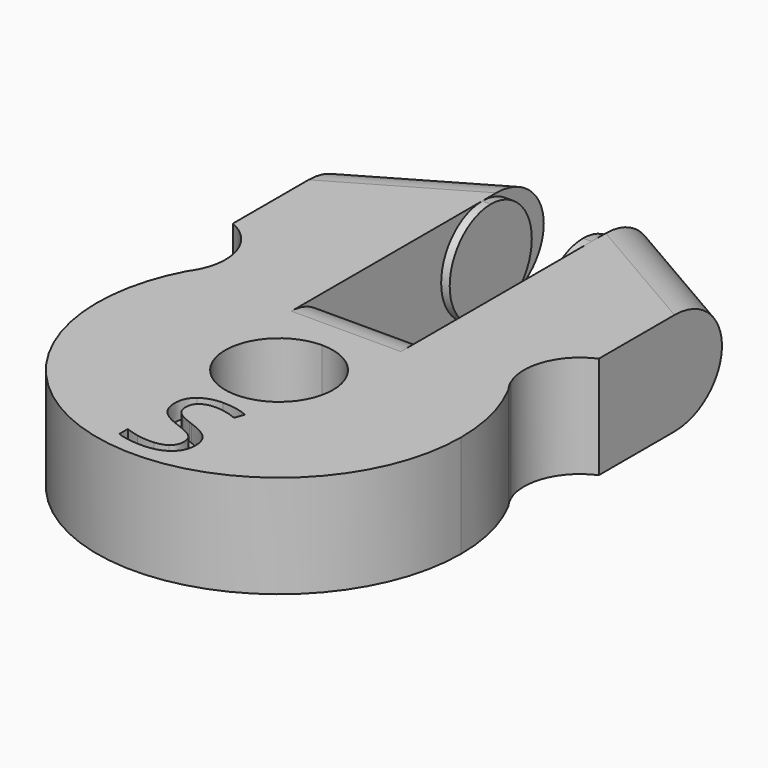
from build123d import *

# Parameters (mm, degrees)
F1_DEPTH      = 6
F3_DEPTH      = 0.5
F5_DEPTH      = 0.5
F6_R          = 2.99999
F7_R          = 2.99999
F9_DEPTH      = 1
F10_TEXT_SIZE = 7.638922447
F11_DEPTH     = 1


# Not quite as in the source:
# - a fillet or chamfer is up to 0.001 mm smaller than in the source, because OpenCascade refuses the exact size
# - Text() gives the source's letters only with a copy of the font that has no kerning and outlines rounded to 1/6400 em; it was checked with that copy


with BuildPart() as f1:
    # F0 (on Top) → F1 (new body)
    with BuildSketch(Plane.XY):
        with BuildLine():
            ThreePointArc((-21.257927263, 3.0925971456), (-19.5135237331, 1.2849088277), (-19.5663380414, -1.2266427602))
            ThreePointArc((-19.5663380414, -1.2266427602), (-17.0596555887, 1.5276447909), (-13.757927263, 3.2504758611))
            Line((-13.757927263, 3.2504758611), (-13.757927263, 16.4425971456))
            Line((-13.757927263, 16.4425971456), (-21.257927263, 12.0925971456))
            Line((-21.257927263, 12.0925971456), (-21.257927263, 3.0925971456))
        make_face()
        with BuildLine():
            ThreePointArc((-19.937029438, -1.8621137259), (-13.1593751133, -17.2347921219), (0.092072737, -6.9074028544))
            ThreePointArc((0.092072737, -6.9074028544), (-0.2305379955, -4.3059550041), (-1.178825088, -1.8621137259))
            ThreePointArc((-1.178825088, -1.8621137259), (-1.3821012217, -1.5548376637), (-1.5495164847, -1.2266427602))
            ThreePointArc((-1.5495164847, -1.2266427602), (-4.0561989374, 1.5276447909), (-7.357927263, 3.2504758611))
            Line((-7.357927263, 3.2504758611), (-7.357927263, 1.1925971456))
            Line((-7.357927263, 1.1925971456), (-7.357927263, 0.9928541258))
            Line((-7.357927263, 0.9928541258), (-10.557927263, 0.9928541258))
            Line((-10.557927263, 0.9928541258), (-13.757927263, 0.9928541258))
            Line((-13.757927263, 0.9928541258), (-13.757927263, 1.1925971456))
            Line((-13.757927263, 1.1925971456), (-13.757927263, 3.2504758611))
            ThreePointArc((-13.757927263, 3.2504758611), (-17.0596555887, 1.5276447909), (-19.5663380414, -1.2266427602))
            ThreePointArc((-19.5663380414, -1.2266427602), (-19.7337533043, -1.5548376637), (-19.937029438, -1.8621137259))
        make_face()
        with BuildLine():
            ThreePointArc((-7.407927263, -6.9074028544), (-12.7853136237, -9.1347892152), (-10.557927263, -3.7574028544))
            ThreePointArc((-10.557927263, -3.7574028544), (-8.3305409023, -4.6800164937), (-7.407927263, -6.9074028544))
        make_face(mode=Mode.SUBTRACT)
        with BuildLine():
            ThreePointArc((-7.357927263, 3.2504758611), (-4.0561989374, 1.5276447909), (-1.5495164847, -1.2266427602))
            ThreePointArc((-1.5495164847, -1.2266427602), (-1.6023307929, 1.2849088277), (0.142072737, 3.0925971456))
            Line((0.142072737, 3.0925971456), (0.142072737, 12.0925971456))
            Line((0.142072737, 12.0925971456), (-7.357927263, 16.4425971456))
            Line((-7.357927263, 16.4425971456), (-7.357927263, 3.2504758611))
        make_face()
    extrude(amount=F1_DEPTH)

    # F2 (on face) → F3 (join)
    with BuildSketch(Plane.YZ.offset(-13.757927263)):
        with BuildLine():
            ThreePointArc((11.9425971456, 0), (14.0639174891, 0.8786796564), (14.9425971456, 3))
            ThreePointArc((14.9425971456, 3), (14.0639174891, 5.1213203436), (11.9425971456, 6))
            ThreePointArc((11.9425971456, 6), (8.9425971456, 3), (11.9425971456, 0))
        make_face()
    extrude(amount=F3_DEPTH)

    # F4 (on face) → F5 (join)
    with BuildSketch(Plane(origin=(-7.357927263, 0, 0), x_dir=(0, -1, 0), z_dir=(-1, 0, 0))):
        with BuildLine():
            ThreePointArc((-11.9425971456, 0), (-9.821276802, 0.8786796564), (-8.9425971456, 3))
            ThreePointArc((-8.9425971456, 3), (-9.821276802, 5.1213203436), (-11.9425971456, 6))
            ThreePointArc((-11.9425971456, 6), (-14.9425971456, 3), (-11.9425971456, 0))
        make_face()
    extrude(amount=F5_DEPTH)

    # F6 (radius 3 in the source; OpenCascade refuses exactly that, so slightly less here)
    f6_edges = [f1.edges().sort_by_distance(p)[0] for p in [
        (-10.557927, 0.992854, 0),
        (-10.557927, 0.992854, 6),
    ]]
    fillet(f6_edges, radius=F6_R)

    # F7 (radius 3 in the source; OpenCascade refuses exactly that, so slightly less here)
    f7_edges = [f1.edges().sort_by_distance(p)[0] for p in [
        (-3.607927, 14.267597, 6),
        (-3.607927, 14.267597, 0),
        (-17.507927, 14.267597, 6),
        (-17.507927, 14.267597, 0),
    ]]
    fillet(f7_edges, radius=F7_R)

    # F8 (on face) → F9 (cut)
    with BuildSketch(Plane.XY.offset(6)):
        with BuildLine():
            add(Edge.make_bspline(
                [(-10.5501950657, -13.4776108282), (-10.4694705412, -13.508341298), (-10.3808423724, -13.5400237976)],
                knots=[0.8265090997, 0.8265090997, 0.8265090997, 1, 1, 1], degree=2))
            Line((-10.5501950657, -13.4776108282), (-10.5494352835, -14.1232135045))
            add(Edge.make_bspline(
                [(-10.0138167139, -14.3677710958), (-10.2080598556, -14.256092153), (-10.5494352835, -14.1232135045)],
                knots=[0, 0, 0, 0.7281433035, 0.7281433035, 0.7281433035], degree=2))
            add(Edge.make_bspline(
                [(-9.6330648925, -14.7019733214), (-9.747051723, -14.5211460458), (-10.0138167139, -14.3677710958)],
                knots=[0, 0, 0, 1, 1, 1], degree=2))
            add(Edge.make_bspline(
                [(-9.5190780619, -15.1656789096), (-9.5190780619, -14.8828005971), (-9.6330648925, -14.7019733214)],
                knots=[0, 0, 0, 1, 1, 1], degree=2))
            add(Edge.make_bspline(
                [(-9.8401509144, -15.83587373), (-9.5190780619, -15.5953674854), (-9.5190780619, -15.1656789096)],
                knots=[0, 0, 0, 1, 1, 1], degree=2))
            add(Edge.make_bspline(
                [(-10.5471486979, -16.0661725929), (-10.0950786813, -16.0268326334), (-9.8401509144, -15.83587373)],
                knots=[0.2060127012, 0.2060127012, 0.2060127012, 1, 1, 1], degree=2))
            Line((-10.5471486979, -16.0661725929), (-10.5464937488, -16.6226963909))
            add(Edge.make_bspline(
                [(-9.4003169139, -16.2291581348), (-9.840740894, -16.5694171183), (-10.5464937488, -16.6226963909)],
                knots=[0, 0, 0, 0.8434155299, 0.8434155299, 0.8434155299], degree=2))
            add(Edge.make_bspline(
                [(-8.8781259363, -15.1059999407), (-8.8781259363, -15.8257283053), (-9.4003169139, -16.2291581348)],
                knots=[0, 0, 0, 1, 1, 1], degree=2))
            add(Edge.make_bspline(
                [(-9.2003923682, -14.1964924551), (-8.8781259363, -14.5474047921), (-8.8781259363, -15.1059999407)],
                knots=[0, 0, 0, 1, 1, 1], degree=2))
            add(Edge.make_bspline(
                [(-10.3808423724, -13.5400237976), (-9.5226588001, -13.8455801182), (-9.2003923682, -14.1964924551)],
                knots=[0, 0, 0, 1, 1, 1], degree=2))
        make_face()
        with BuildLine():
            Line((-10.5464937488, -16.6226963909), (-10.5471486979, -16.0661725929))
            add(Edge.make_bspline(
                [(-10.7950144164, -16.0763799745), (-10.6644454927, -16.0763799745), (-10.5471486979, -16.0661725929)],
                knots=[0, 0, 0, 0.2060127012, 0.2060127012, 0.2060127012], degree=2))
            add(Edge.make_bspline(
                [(-11.5780024879, -15.9940229975), (-11.182927714, -16.0763799745), (-10.7950144164, -16.0763799745)],
                knots=[0, 0, 0, 1, 1, 1], degree=2))
            add(Edge.make_bspline(
                [(-12.3096666463, -15.7708236539), (-11.9730772618, -15.9116660204), (-11.5780024879, -15.9940229975)],
                knots=[0, 0, 0, 1, 1, 1], degree=2))
            Line((-12.3096666463, -15.7708236539), (-12.3096666463, -16.3819362951))
            add(Edge.make_bspline(
                [(-10.8176924245, -16.6325879644), (-11.786878879, -16.6325879644), (-12.3096666463, -16.3819362951)],
                knots=[0, 0, 0, 1, 1, 1], degree=2))
            add(Edge.make_bspline(
                [(-10.5464937488, -16.6226963909), (-10.6775204288, -16.6325879644), (-10.8176924245, -16.6325879644)],
                knots=[0.8434155299, 0.8434155299, 0.8434155299, 1, 1, 1], degree=2))
        make_face()
        with BuildLine():
            Line((-10.5524124649, -11.5934408654), (-10.5530795319, -11.0266202683))
            add(Edge.make_bspline(
                [(-11.7647976605, -11.3993391842), (-11.3043852206, -11.0364668325), (-10.5530795319, -11.0266202683)],
                knots=[0, 0, 0, 0.9728649367, 0.9728649367, 0.9728649367], degree=2))
            add(Edge.make_bspline(
                [(-12.2380518836, -12.4025426509), (-12.2380518836, -11.7723327396), (-11.7647976605, -11.3993391842)],
                knots=[0, 0, 0, 1, 1, 1], degree=2))
            add(Edge.make_bspline(
                [(-11.9116079239, -13.3759066332), (-12.2380518836, -13.0029130777), (-12.2380518836, -12.4025426509)],
                knots=[0, 0, 0, 1, 1, 1], degree=2))
            add(Edge.make_bspline(
                [(-10.8248539008, -14.0210362866), (-11.5851639642, -13.7489001886), (-11.9116079239, -13.3759066332)],
                knots=[0, 0, 0, 1, 1, 1], degree=2))
            add(Edge.make_bspline(
                [(-10.5494352835, -14.1232135045), (-10.6768898596, -14.0736024592), (-10.8248539008, -14.0210362866)],
                knots=[0.7281433035, 0.7281433035, 0.7281433035, 1, 1, 1], degree=2))
            Line((-10.5494352835, -14.1232135045), (-10.5501950657, -13.4776108282))
            add(Edge.make_bspline(
                [(-11.1399588564, -13.2064183616), (-10.9347659794, -13.331211145), (-10.5501950657, -13.4776108282)],
                knots=[0, 0, 0, 0.8265090997, 0.8265090997, 0.8265090997], degree=2))
            add(Edge.make_bspline(
                [(-11.4926615624, -12.874006505), (-11.3882233669, -13.0554305703), (-11.1399588564, -13.2064183616)],
                knots=[0, 0, 0, 1, 1, 1], degree=2))
            add(Edge.make_bspline(
                [(-11.597099758, -12.4097041272), (-11.597099758, -12.6925824396), (-11.4926615624, -12.874006505)],
                knots=[0, 0, 0, 1, 1, 1], degree=2))
            add(Edge.make_bspline(
                [(-11.3136246558, -11.8093337003), (-11.597099758, -12.0253715676), (-11.597099758, -12.4097041272)],
                knots=[0, 0, 0, 1, 1, 1], degree=2))
            add(Edge.make_bspline(
                [(-10.5524124649, -11.5934408654), (-11.0374943946, -11.598893375), (-11.3136246558, -11.8093337003)],
                knots=[0.0259100037, 0.0259100037, 0.0259100037, 1, 1, 1], degree=2))
        make_face()
        with BuildLine():
            add(Edge.make_bspline(
                [(-10.5530795319, -11.0266202683), (-10.5321241797, -11.0263456288), (-10.5109425245, -11.0263456288)],
                knots=[0.9728649367, 0.9728649367, 0.9728649367, 1, 1, 1], degree=2))
            Line((-10.5530795319, -11.0266202683), (-10.5524124649, -11.5934408654))
            add(Edge.make_bspline(
                [(-10.5264590564, -11.593295833), (-10.5395096791, -11.593295833), (-10.5524124649, -11.5934408654)],
                knots=[0, 0, 0, 0.0259100037, 0.0259100037, 0.0259100037], degree=2))
            add(Edge.make_bspline(
                [(-9.2135217413, -11.8761741455), (-9.8890876689, -11.593295833), (-10.5264590564, -11.593295833)],
                knots=[0, 0, 0, 1, 1, 1], degree=2))
            Line((-9.2135217413, -11.8761741455), (-9.0153875647, -11.3247404731))
            add(Edge.make_bspline(
                [(-10.5109425245, -11.0263456288), (-9.6981149685, -11.0263456288), (-9.0153875647, -11.3247404731)],
                knots=[0, 0, 0, 1, 1, 1], degree=2))
        make_face()
    extrude(amount=-F9_DEPTH, mode=Mode.SUBTRACT)

    # F10 (on face) → F11 (cut)
    with BuildSketch(Plane(origin=(0, 0, 0), x_dir=(1, 0, 0), z_dir=(0, 0, -1))):
        with Locations((-12.7047455028, 11.0573786926)):
            Text('S', F10_TEXT_SIZE, font='Open Sans', text_align=(TextAlign.LEFT, TextAlign.BOTTOM))
    extrude(amount=-F11_DEPTH, mode=Mode.SUBTRACT)


solid = f1.part
